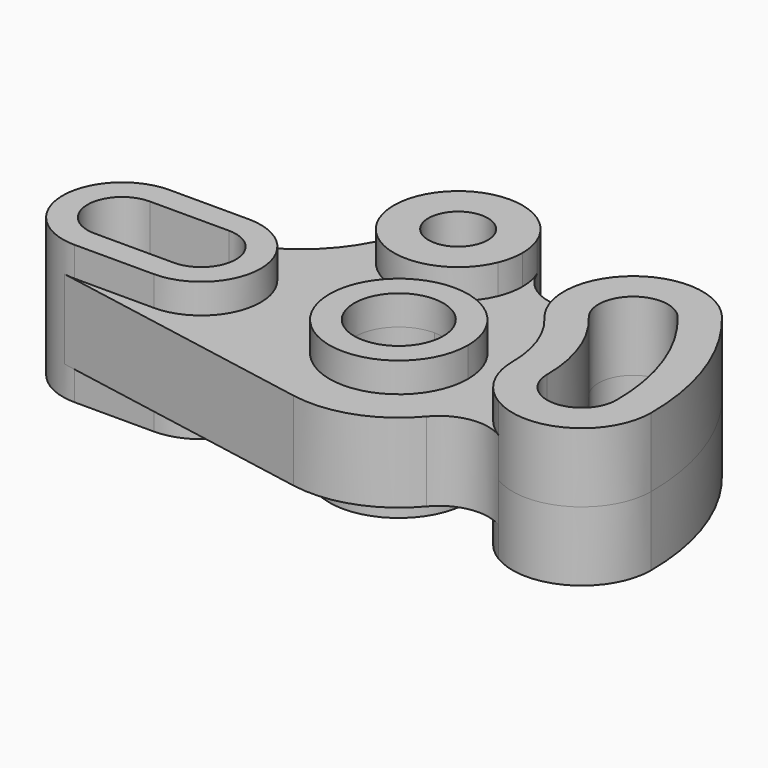
from build123d import *

# Parameters (mm, degrees)
F1_DEPTH = 12.7
F0_R     = 9.525
F2_DEPTH = 22.225


with BuildPart() as f1:
    # F0 (on Top) → F1 (new body, symmetric)
    with BuildSketch(Plane.XY):
        with BuildLine():
            ThreePointArc((88.7222, 14.2875), (98.8249881362, 10.1027881362), (103.0097, 0))
            Line((103.0097, 0), (110.9472, 0))
            ThreePointArc((110.9472, 0), (104.4376482119, 15.7154482119), (88.7222, 22.225))
            Line((88.7222, 22.225), (88.7222, 14.2875))
        make_face()
        with BuildLine():
            Line((66.4972, 0), (74.4347, 0))
            ThreePointArc((74.4347, 0), (78.6194118638, 10.1027881362), (88.7222, 14.2875))
            Line((88.7222, 14.2875), (88.7222, 22.225))
            ThreePointArc((88.7222, 22.225), (73.0067517881, 15.7154482119), (66.4972, 0))
        make_face()
        with BuildLine():
            ThreePointArc((88.7222, 22.225), (104.4376482119, 15.7154482119), (110.9472, 0))
            Line((110.9472, 0), (125.222, 0))
            ThreePointArc((125.222, 0), (123.0207927202, 12.4836668274), (116.682668965, 23.461619196))
            ThreePointArc((116.682668965, 23.461619196), (111.4870759361, 37.3222969765), (116.1485113735, 51.3716241887))
            ThreePointArc((116.1485113735, 51.3716241887), (101.3767802444, 45.3853872913), (88.852182223, 55.2430501556))
            ThreePointArc((88.852182223, 55.2430501556), (89.9420456997, 51.5031131444), (90.3097, 47.625))
            ThreePointArc((90.3097, 47.625), (89.9089336946, 43.5776532611), (88.7222, 39.6875))
            Line((88.7222, 39.6875), (88.7222, 22.225))
        make_face()
        with BuildLine():
            Line((125.222, 0), (110.9472, 0))
            ThreePointArc((110.9472, 0), (88.7222, -22.225), (66.4972, 0))
            Line((66.4972, 0), (44.45, 0))
            ThreePointArc((44.45, 0), (38.8703841816, -13.4703841816), (25.4, -19.05))
            Line((25.4, -19.05), (0, -19.05))
            ThreePointArc((0, -19.05), (-1.7112193853, -18.9729868027), (-3.4086029201, -18.7425698914))
            Line((-3.4086029201, -18.7425698914), (82.4730946464, -34.3613781342))
            ThreePointArc((82.4730946464, -34.3613781342), (100.6094978328, -32.8397286109), (115.5177113754, -22.3999150697))
            ThreePointArc((115.5177113754, -22.3999150697), (125.0932774359, -16.9217551289), (135.9264520761, -19.005988544))
            ThreePointArc((135.9264520761, -19.005988544), (128.0821503671, -10.9065679155), (125.222, 0))
        make_face()
        with BuildLine():
            Line((44.45, 0), (66.4972, 0))
            ThreePointArc((66.4972, 0), (73.0067517881, 15.7154482119), (88.7222, 22.225))
            Line((88.7222, 22.225), (88.7222, 39.6875))
            ThreePointArc((88.7222, 39.6875), (63.1687863903, 28.0389841297), (49.6579571791, 52.6585365854))
            ThreePointArc((49.6579571791, 52.6585365854), (33.8807382573, 28.4450035745), (6.5503572572, 19.05))
            Line((6.5503572572, 19.05), (25.4, 19.05))
            ThreePointArc((25.4, 19.05), (38.8703841816, 13.4703841816), (44.45, 0))
        make_face()
    extrude(amount=F1_DEPTH, both=True)

    # F0 (on Top) → F2 (join, symmetric)
    with BuildSketch(Plane.XY):
        with BuildLine():
            ThreePointArc((88.7222, 14.2875), (98.8249881362, 10.1027881362), (103.0097, 0))
            Line((103.0097, 0), (110.9472, 0))
            ThreePointArc((110.9472, 0), (104.4376482119, 15.7154482119), (88.7222, 22.225))
            Line((88.7222, 22.225), (88.7222, 14.2875))
        make_face()
        with BuildLine():
            Line((110.9472, 0), (103.0097, 0))
            ThreePointArc((103.0097, 0), (88.7222, -14.2875), (74.4347, 0))
            Line((74.4347, 0), (66.4972, 0))
            ThreePointArc((66.4972, 0), (88.7222, -22.225), (110.9472, 0))
        make_face()
        with BuildLine():
            Line((66.4972, 0), (74.4347, 0))
            ThreePointArc((74.4347, 0), (78.6194118638, 10.1027881362), (88.7222, 14.2875))
            Line((88.7222, 14.2875), (88.7222, 22.225))
            ThreePointArc((88.7222, 22.225), (73.0067517881, 15.7154482119), (66.4972, 0))
        make_face()
        with BuildLine():
            ThreePointArc((116.682668965, 23.461619196), (123.0207927202, 12.4836668274), (125.222, 0))
            Line((125.222, 0), (136.3218, 0))
            ThreePointArc((136.3218, 0), (133.4511928724, 16.2800220142), (125.1856090747, 30.596433106))
            ThreePointArc((125.1856090747, 30.596433106), (126.556865998, 46.2699714599), (142.2304043519, 44.8987145366))
            ThreePointArc((142.2304043519, 44.8987145366), (154.3597295619, 23.8901070113), (158.5722, 0))
            Line((158.5722, 0), (169.672, 0))
            ThreePointArc((169.672, 0), (164.7901297141, 27.6864621982), (150.7333444616, 52.0335284466))
            ThreePointArc((150.7333444616, 52.0335284466), (133.2827298684, 59.9685045985), (116.1485113735, 51.3716241887))
            ThreePointArc((116.1485113735, 51.3716241887), (111.4870759361, 37.3222969765), (116.682668965, 23.461619196))
        make_face()
        with BuildLine():
            Line((136.3218, 0), (125.222, 0))
            ThreePointArc((125.222, 0), (128.0821503671, -10.9065679155), (135.9264520761, -19.005988544))
            ThreePointArc((135.9264520761, -19.005988544), (158.3535679155, -19.3648496329), (169.672, 0))
            Line((169.672, 0), (158.5722, 0))
            ThreePointArc((158.5722, 0), (147.447, -11.1252), (136.3218, 0))
        make_face()
        with BuildLine():
            ThreePointArc((25.4, -19.05), (38.8703841816, -13.4703841816), (44.45, 0))
            ThreePointArc((44.45, 0), (38.8703841816, 13.4703841816), (25.4, 19.05))
            Line((25.4, 19.05), (6.5503572572, 19.05))
            Line((6.5503572572, 19.05), (0, 19.05))
            ThreePointArc((0, 19.05), (-18.9729868027, 1.7112193853), (-3.4086029201, -18.7425698914))
            ThreePointArc((-3.4086029201, -18.7425698914), (-1.7112193853, -18.9729868027), (0, -19.05))
            Line((0, -19.05), (25.4, -19.05))
        make_face()
        with BuildLine():
            ThreePointArc((25.4, 11.0998), (33.2487438498, 7.8487438498), (36.4998, 0))
            ThreePointArc((36.4998, 0), (33.2487438498, -7.8487438498), (25.4, -11.0998))
            Line((25.4, -11.0998), (0, -11.0998))
            ThreePointArc((0, -11.0998), (-11.0998, 0), (0, 11.0998))
            Line((0, 11.0998), (25.4, 11.0998))
        make_face(mode=Mode.SUBTRACT)
        with BuildLine():
            ThreePointArc((49.6579571791, 52.6585365854), (63.1687863903, 28.0389841297), (88.7222, 39.6875))
            ThreePointArc((88.7222, 39.6875), (89.9089336946, 43.5776532611), (90.3097, 47.625))
            ThreePointArc((90.3097, 47.625), (89.9420456997, 51.5031131444), (88.852182223, 55.2430501556))
            ThreePointArc((88.852182223, 55.2430501556), (68.314287895, 68.217777398), (49.6579571791, 52.6585365854))
        make_face()
        with Locations((69.6722, 47.625)):
            Circle(F0_R, mode=Mode.SUBTRACT)
    extrude(amount=F2_DEPTH, both=True)


solid = f1.part
